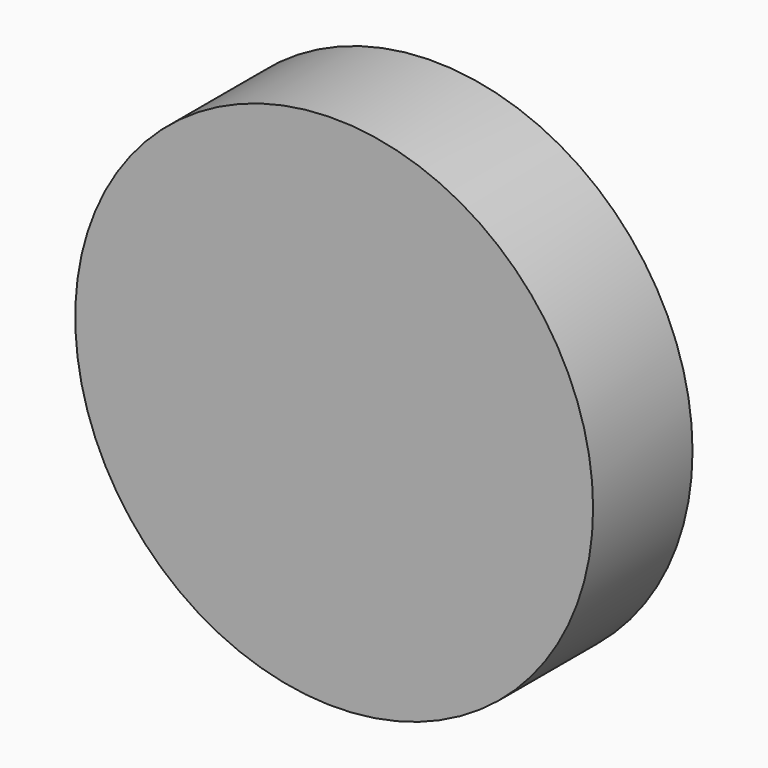
from build123d import *

# Parameters (mm, degrees)
F0_R     = 25
F1_DEPTH = 12


# Not quite as in the source:
# - the program builds the solid bodies; features that only make, move or delete a surface that nothing else refers to are left out


with BuildPart() as f1:
    # F0 (on Front) → F1 (new body)
    with BuildSketch(Plane.XZ):
        Circle(F0_R)
    extrude(amount=F1_DEPTH)


solid = f1.part
